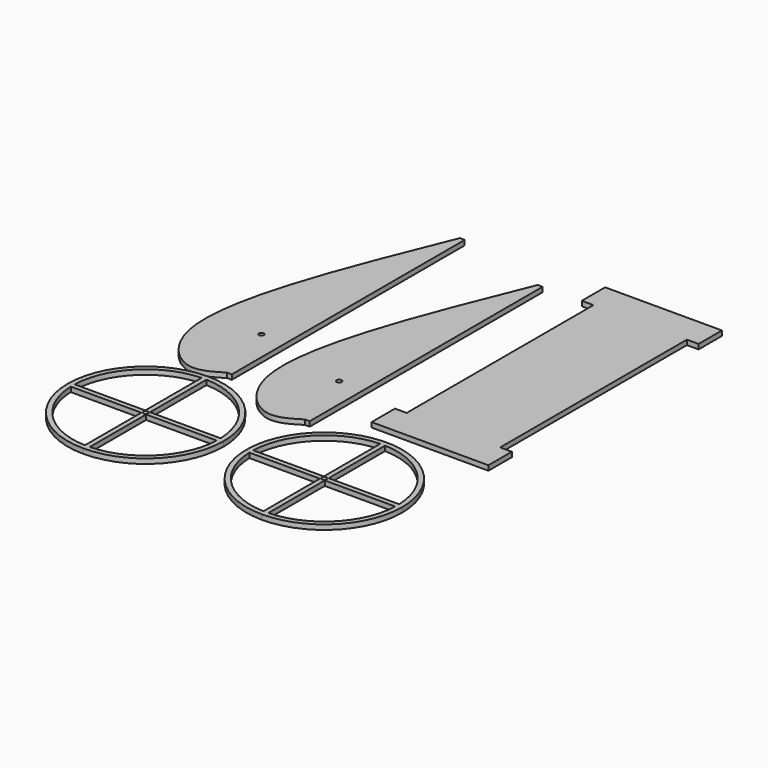
from build123d import *

# Parameters (mm, degrees)
F0_R     = 1.651
F1_DEPTH = 3.175


# Not quite as in the source:
# - a feature names something its author has since deleted; it is built from what else it names


with BuildPart() as f1:
    # F0 (on Top) → F1 (new body)
    with BuildSketch(Plane.XY):
        with BuildLine():
            ThreePointArc((65.7106608197, -101.6), (-21.0103637537, -65.6789756049), (14.9106610719, -152.4))
            ThreePointArc((14.9106610719, -152.4), (50.8316853932, -137.5210243951), (65.7106608197, -101.6))
        make_face()
        with BuildLine():
            Line((-32.6878734933, -103.1875), (13.3231608197, -103.1875))
            Line((13.3231608197, -103.1875), (13.3231608197, -149.198534313))
            ThreePointArc((13.3231608197, -149.198534313), (-18.7652996343, -135.275960454), (-32.6878734933, -103.1875))
        make_face(mode=Mode.SUBTRACT)
        with BuildLine():
            Line((13.3231608197, -54.001465687), (13.3231608197, -100.0126722037))
            Line((13.3231608197, -100.0126722037), (-32.6878792363, -100.0126722037))
            ThreePointArc((-32.6878792363, -100.0126722037), (-18.7653605513, -67.9241004631), (13.3231608197, -54.001465687))
        make_face(mode=Mode.SUBTRACT)
        with BuildLine():
            ThreePointArc((62.5091951328, -103.1875), (48.5855888423, -135.2769928537), (16.4952423273, -149.1986315606))
            Line((16.4952423273, -149.1986315606), (16.4952423273, -103.1875))
            Line((16.4952423273, -103.1875), (62.5091951328, -103.1875))
        make_face(mode=Mode.SUBTRACT)
        with Locations((14.9106608197, -101.6)):
            Circle(F0_R, mode=Mode.SUBTRACT)
        with BuildLine():
            Line((16.4952423273, -100.0126722037), (16.4952423273, -54.0013684394))
            ThreePointArc((16.4952423273, -54.0013684394), (48.5856497612, -67.9230680615), (62.5092008758, -100.0126722037))
            Line((62.5092008758, -100.0126722037), (16.4952423273, -100.0126722037))
        make_face(mode=Mode.SUBTRACT)
    extrude(amount=F1_DEPTH)


with BuildPart() as f1b:
    # F0 (on Top) → F1, piece 2 (new body)
    with BuildSketch(Plane.XY):
        with BuildLine():
            ThreePointArc((-152.4, -101.6), (-137.5210244843, -137.5210244843), (-101.6, -152.4))
            ThreePointArc((-101.6, -152.4), (-65.6789755157, -137.5210244843), (-50.8, -101.6))
            ThreePointArc((-50.8, -101.6), (-101.6, -50.8), (-152.4, -101.6))
        make_face()
        with BuildLine():
            Line((-149.198534313, -103.1875), (-103.1875, -103.1875))
            Line((-103.1875, -103.1875), (-103.1875, -149.198534313))
            ThreePointArc((-103.1875, -149.198534313), (-135.275960454, -135.275960454), (-149.198534313, -103.1875))
        make_face(mode=Mode.SUBTRACT)
        with BuildLine():
            Line((-103.1875, -54.001465687), (-103.1875, -100.0126722037))
            Line((-103.1875, -100.0126722037), (-149.198540056, -100.0126722037))
            ThreePointArc((-149.198540056, -100.0126722037), (-135.276021371, -67.9241004631), (-103.1875, -54.001465687))
        make_face(mode=Mode.SUBTRACT)
        with Locations((-101.6, -101.6)):
            Circle(F0_R, mode=Mode.SUBTRACT)
        with BuildLine():
            ThreePointArc((-54.001465687, -103.1875), (-67.9250719774, -135.2769928537), (-100.0154184924, -149.1986315606))
            Line((-100.0154184924, -149.1986315606), (-100.0154184924, -103.1875))
            Line((-100.0154184924, -103.1875), (-54.001465687, -103.1875))
        make_face(mode=Mode.SUBTRACT)
        with BuildLine():
            Line((-100.0154184924, -100.0126722037), (-100.0154184924, -54.0013684394))
            ThreePointArc((-100.0154184924, -54.0013684394), (-67.9250110585, -67.9230680615), (-54.001459944, -100.0126722037))
            Line((-54.001459944, -100.0126722037), (-100.0154184924, -100.0126722037))
        make_face(mode=Mode.SUBTRACT)
    extrude(amount=F1_DEPTH)


with BuildPart() as f1c:
    # F0 (on Top) → F1, piece 3 (new body)
    with BuildSketch(Plane.XY):
        Polygon((71.12, 133.35), (71.12, 152.4), (-5.08, 152.4), (-5.08, 133.35), (2.54, 133.35), (2.54, -18.9738), (-5.08, -18.9738), (-5.08, -38.0238), (71.12, -38.0238), (71.12, -18.9738), (63.5, -18.9738), (63.5, 133.35), align=None)
    extrude(amount=F1_DEPTH)


with BuildPart() as f1d:
    # F0 (on Top) → F1, piece 4 (new body)
    with BuildSketch(Plane.XY):
        with BuildLine():
            Line((-93.6064264297, 148.5900000185), (-96.7814264297, 148.5900000185))
            add(Edge.make_bspline(
                [(-96.7814264297, 148.5900000185), (-122.8968017051, 84.5413605912), (-161.6813226062, -10.5786891249), (-117.4032009161, -54.2310342357), (-102.8189814093, -45.1346689408), (-96.7814264297, -41.3689682424)],
                knots=[0, 0, 0, 0, 0.5470988668, 0.8125086166, 1, 1, 1, 1], degree=3))
            Line((-96.7814264297, -41.3689682424), (-93.6064264297, -41.3689682424))
            Line((-93.6064264297, -41.3689682424), (-93.6064264297, 148.5900000185))
        make_face()
        with Locations((-109.4814264297, 2.5445778297)):
            Circle(F0_R, mode=Mode.SUBTRACT)
    extrude(amount=F1_DEPTH)


with BuildPart() as f1e:
    # F0 (on Top) → F1, piece 5 (new body)
    with BuildSketch(Plane.XY):
        with BuildLine():
            Line((-30.3171201937, 132.9683979097), (-33.4921201937, 132.9683979097))
            add(Edge.make_bspline(
                [(-33.4921201937, 132.9683979097), (-59.6074954691, 68.9197584825), (-98.3920163702, -26.2002912337), (-54.1195029261, -69.8471073591), (-39.5378329238, -60.761356619), (-33.504356178, -56.9982020903)],
                knots=[0, 0, 0, 0, 0.5470988668, 0.8125086166, 0.9998733405, 0.9998733405, 0.9998733405, 0.9998733405], degree=3))
            Line((-33.504356178, -56.9982020903), (-30.3171201937, -56.9982020903))
            Line((-30.3171201937, -56.9982020903), (-30.3171201937, 132.9683979097))
        make_face()
        with Locations((-46.1921201937, -13.0816020903)):
            Circle(F0_R, mode=Mode.SUBTRACT)
    extrude(amount=F1_DEPTH)


solid = Compound([f1.part, f1b.part, f1c.part, f1d.part, f1e.part])
